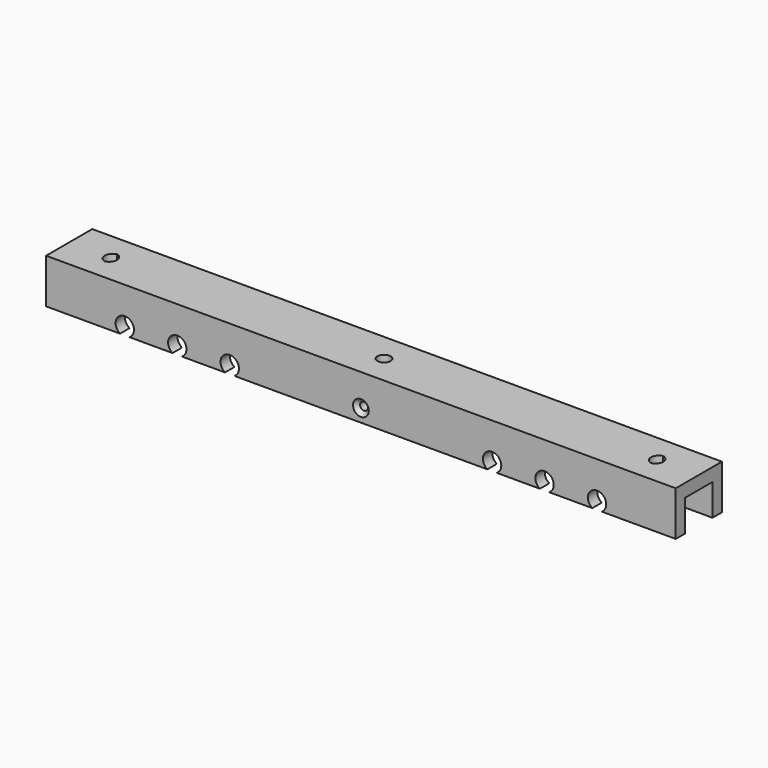
from build123d import *

# Parameters (mm, degrees)
F0_W            = 120
F0_H            = 2.25
F0_H_2          = 6.5
F1_DEPTH        = 2.5
F2_DEPTH        = 6
F6_D            = 3
F6_CSINK_D      = 5
F6_CSINK_ANGLE  = 90
F7_D            = 2.5
F8_D            = 3.5
F8_DEPTH        = 3
F8_TIP          = 1.0515060833
F10_D           = 1.5
F10_CSINK_D     = 3
F10_CSINK_ANGLE = 90


# Not quite as in the source:
# - a feature names something its author has since deleted; it is built from what else it names


with BuildPart() as f1:
    # F0 (on Top) → F1 (new body)
    with BuildSketch(Plane.XY):
        with Locations((0, 4.375)):
            Rectangle(F0_W, F0_H)
        Rectangle(F0_W, F0_H_2)
        with Locations((0, -4.375)):
            Rectangle(F0_W, F0_H)
    extrude(amount=F1_DEPTH)

    # F0 (on Top) → F2 (join)
    with BuildSketch(Plane.XY):
        with Locations((0, 4.375)):
            Rectangle(F0_W, F0_H)
        with Locations((0, -4.375)):
            Rectangle(F0_W, F0_H)
    extrude(amount=-F2_DEPTH)

    # F6 (through all)
    with Locations(Plane(origin=(0, 0, 0), x_dir=(1, 0, 0), z_dir=(0, 0, -1))):
        with Locations((-52.377641201, 0), (51.710255444, 0)):
            CounterSinkHole(F6_D / 2, F6_CSINK_D / 2, counter_sink_angle=F6_CSINK_ANGLE)

    # F7 (through all)
    with Locations(Plane(origin=(0, 0, 0), x_dir=(1, 0, 0), z_dir=(0, 0, -1))):
        with Locations((0, 0)):
            Hole(F7_D / 2)

    # F8
    with Locations(Plane.XZ.offset(5.5)):
        with Locations((-45, -4.5), (-35, -4.5), (-25, -4.5), (25, -4.5), (35, -4.5), (45, -4.5)):
            Hole(F8_D / 2, depth=F8_DEPTH)
            with Locations((0, 0, -(F8_DEPTH + F8_TIP / 2))):  # 118° drill point
                Cone(0, F8_D / 2, F8_TIP, mode=Mode.SUBTRACT)

    # F10 (through all)
    with Locations(Plane.XZ.offset(5.5)):
        with Locations((0, -3.5449948628)):
            CounterSinkHole(F10_D / 2, F10_CSINK_D / 2, counter_sink_angle=F10_CSINK_ANGLE)

    # F11: F1 across plane


with BuildPart() as f1_1:
    add(f1.part)
    add(f1.part.mirror(Plane.YZ))


solid = f1_1.part
